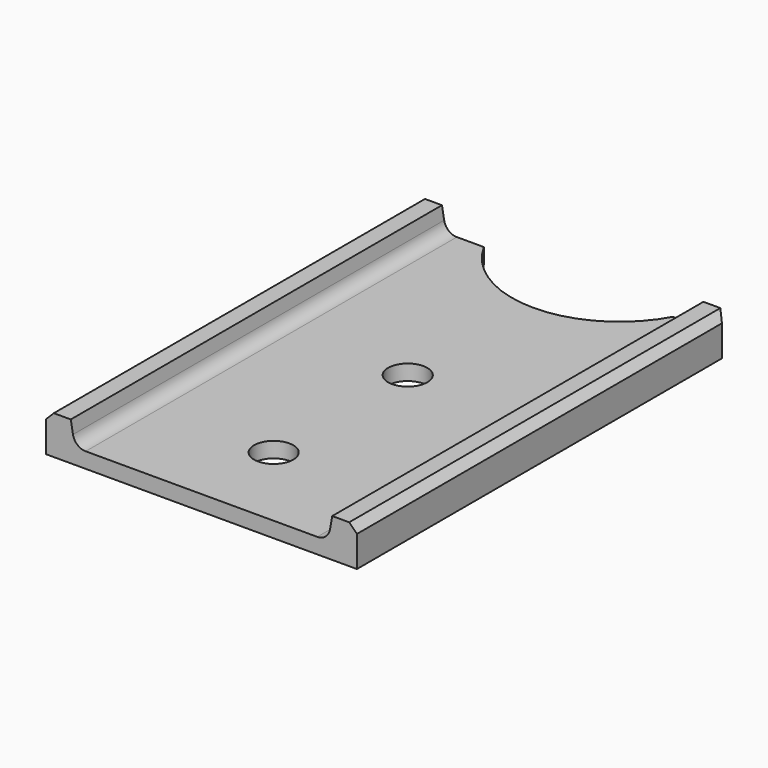
from build123d import *

# Parameters (mm, degrees)
F1_DEPTH = 228.6
F2_SIZE  = 3.81
F4_DEPTH = 25.4
F5_R     = 9.652
F6_DEPTH = 25.4


# Not quite as in the source:
# - a feature names something its author has since deleted; it is built from what else it names


with BuildPart() as f1:
    # F0 (on Front) → F1 (new body)
    with BuildSketch(Plane.XZ):
        with BuildLine():
            Line((-168.0421057219, 19.05), (-168.0421057219, 0))
            Line((-168.0421057219, 0), (-14.8801057219, 0))
            Line((-14.8801057219, 0), (-14.8801057219, 19.05))
            Line((-14.8801057219, 19.05), (-27.0467057219, 19.05))
            Line((-27.0467057219, 19.05), (-28.1368765378, 12.8673340718))
            ThreePointArc((-28.1368765378, 12.8673340718), (-30.3108938413, 9.1037793136), (-34.3961226724, 7.62))
            Line((-34.3961226724, 7.62), (-91.4611057219, 7.62))
            Line((-91.4611057219, 7.62), (-148.5260887714, 7.62))
            ThreePointArc((-148.5260887714, 7.62), (-152.6077900929, 9.1056177862), (-154.7796180031, 12.8673340718))
            Line((-154.7796180031, 12.8673340718), (-155.8697888189, 19.05))
            Line((-155.8697888189, 19.05), (-168.0421057219, 19.05))
        make_face()
    extrude(amount=F1_DEPTH)

    # F2
    f2_edges = [f1.edges().sort_by_distance(p)[0] for p in [
        (-168.042106, -114.3, 19.05),
        (-14.880106, -114.3, 19.05),
        (-14.880106, 0, 9.525),
        (-168.042106, 0, 9.525),
    ]]
    chamfer(f2_edges, length=F2_SIZE)

    # F3 (on face) → F4 (cut)
    with BuildSketch(Plane.XY.offset(7.62)):
        with BuildLine():
            Line((-42.1433808409, 0), (-135.2288363374, 0))
            ThreePointArc((-135.2288363374, 0), (-88.6861085892, -27.6225), (-42.1433808409, 0))
        make_face()
    extrude(amount=-F4_DEPTH, mode=Mode.SUBTRACT)

    # F5 (on face) → F6 (cut)
    with BuildSketch(Plane(origin=(0, 0, 0), x_dir=(1, 0, 0), z_dir=(0, 0, -1))):
        with Locations((-91.4611057219, 101.6)):
            Circle(F5_R)
        with Locations((-91.4611057219, 184.15)):
            Circle(F5_R)
    extrude(amount=-F6_DEPTH, mode=Mode.SUBTRACT)


solid = f1.part
